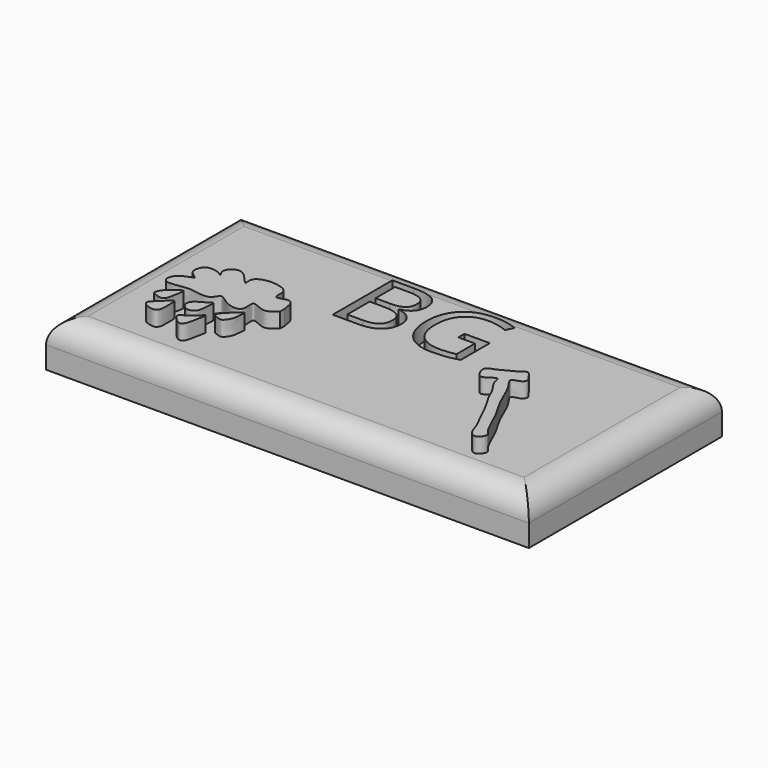
from build123d import *
from build123d import SkipClean  # not in build123d's __all__

# Parameters (mm, degrees)
F0_W         = 101.6
F0_H         = 50.8
F1_DEPTH     = 9.525
F2_TEXT_SIZE = 21.9851628774
F3_DEPTH     = 3.556
F4_T1_DEPTH  = 126.1284097937
F4_T3_DEPTH  = 75.3284097937
F6_DEPTH     = 3.175
F8_DEPTH     = 3.175


# Not quite as in the source:
# - a fillet or chamfer that OpenCascade refuses, or shapes differently, is made with other operations: its cross-section is extruded or revolved along the edge and cut away or added
# - Text() gives the source's letters only with a copy of the font that has no kerning and outlines rounded to 1/6400 em; it was checked with that copy


with BuildPart() as f1:
    # F0 (on Top) → F1 (new body)
    with BuildSketch(Plane.XY):
        with Locations((4.0292814374, -12.5215539605)):
            Rectangle(F0_W, F0_H)
    extrude(amount=F1_DEPTH)

    # F2 (on face) → F3 (cut)
    with BuildSketch(Plane.XY.offset(9.525)):
        with Locations((-12.9512567073, -7.48295011)):
            Text('BG', F2_TEXT_SIZE, font='Open Sans', text_align=(TextAlign.LEFT, TextAlign.BOTTOM))
    extrude(amount=-F3_DEPTH, mode=Mode.SUBTRACT)

    # F4: fillet of radius 4.9056819587 on 4 edges, made by hand

    # F4_s2 → F4_t1 (cut)
    with BuildSketch(Plane.YZ.offset(-59.0349234595)):
        with BuildLine():
            ThreePointArc((-33.0158720017, 9.525), (-36.4847129811, 8.0881590206), (-37.9215539605, 4.6193180413))
            Line((-37.9215539605, 4.6193180413), (-37.9215539605, 9.525))
            Line((-37.9215539605, 9.525), (-33.0158720017, 9.525))
        make_face()
        with BuildLine():
            ThreePointArc((12.8784460395, 4.6193180413), (11.4416050602, 8.0881590206), (7.9727640808, 9.525))
            Line((7.9727640808, 9.525), (12.8784460395, 9.525))
            Line((12.8784460395, 9.525), (12.8784460395, 4.6193180413))
        make_face()
    with SkipClean():  # cleaning this boolean's faces spoils the solid; the shape is the same uncleaned
        extrude(amount=F4_T1_DEPTH, mode=Mode.SUBTRACT)

    # F4_s4 → F4_t3 (cut)
    with BuildSketch(Plane.XZ.offset(-25.1426509364)):
        with BuildLine():
            ThreePointArc((-46.7707185626, 4.6193180413), (-45.3338775832, 8.0881590206), (-41.8650366039, 9.525))
            Line((-41.8650366039, 9.525), (-46.7707185626, 9.525))
            Line((-46.7707185626, 9.525), (-46.7707185626, 4.6193180413))
        make_face()
        with BuildLine():
            ThreePointArc((54.8292814374, 4.6193180413), (53.392440458, 8.0881590206), (49.9235994787, 9.525))
            Line((49.9235994787, 9.525), (54.8292814374, 9.525))
            Line((54.8292814374, 9.525), (54.8292814374, 4.6193180413))
        make_face()
    extrude(amount=F4_T3_DEPTH, mode=Mode.SUBTRACT)

    # F5 (on face) → F6 (join)
    with BuildSketch(Plane.XY.offset(9.525)):
        with BuildLine():
            add(Edge.make_bspline(
                [(-30.1943253726, -12.7980159596), (-30.6638978838, -12.4954709679), (-31.6267253046, -11.8751224446), (-33.7515961581, -11.8213043742), (-34.4176454887, -12.7555614994), (-35.0145429939, -14.6379553372), (-33.6110185049, -15.5878595592), (-32.8381694853, -16.1109231412)],
                knots=[0, 0, 0, 0, 0.2003103356, 0.4107231134, 0.5669213347, 0.7615257699, 1, 1, 1, 1], degree=3))
            add(Edge.make_bspline(
                [(-32.8381694853, -16.1109231412), (-34.112950811, -16.5650307283), (-36.3264014889, -17.3535147812), (-36.5745988024, -20.6952249655), (-32.187577032, -19.7435687353), (-30.2242086338, -19.7475381146), (-26.3365262633, -20.6465069984), (-25.6376160227, -17.6651790254), (-23.2611312044, -20.2929673205), (-18.9913074877, -20.8552925245), (-20.5214901929, -16.0086354704), (-16.807287616, -18.8934549791), (-15.2516189291, -17.4785744542), (-14.4576687431, -16.7564768344)],
                knots=[0, 0, 0, 0, 0.1039781038, 0.1805410855, 0.2831417982, 0.3686725312, 0.4687259635, 0.5411456275, 0.6322911283, 0.7284193522, 0.8168783892, 0.9065421589, 1, 1, 1, 1], degree=3))
            Line((-14.4576687431, -16.7564768344), (-14.4576687431, -15.6208071858))
            add(Edge.make_bspline(
                [(-14.4576687431, -15.6208071858), (-14.6337982566, -14.3014323106), (-14.9696347652, -11.7857025918), (-18.9198891467, -14.113561209), (-17.8391791134, -10.4525662659), (-20.7394672952, -9.4640154529), (-23.252574533, -9.3869308074), (-25.7056960807, -10.5400759818), (-24.7198852466, -13.3743134661), (-27.1734299353, -10.0341195772), (-29.1590570967, -9.1643213191), (-31.2437333359, -11.0235517469), (-30.5359718134, -12.220319388), (-30.1943253726, -12.7980159596)],
                knots=[0, 0, 0, 0, 0.1047918867, 0.1998128573, 0.2885396562, 0.3840489401, 0.4826982162, 0.5732730344, 0.6444100513, 0.7437118311, 0.8326558119, 0.9192206069, 1, 1, 1, 1], degree=3))
        make_face()
        with BuildLine():
            add(Edge.make_bspline(
                [(-22.0946185291, -24.2940131575), (-22.0373505514, -24.6135380633), (-21.0807431356, -24.8821418603), (-19.9589656353, -25.3557262166), (-18.803080228, -23.3856899709), (-18.8393406044, -22.1102220554), (-18.44732324, -20.1385319215), (-20.0988502501, -21.7254314776), (-20.9013918072, -22.4624018961), (-22.1706834832, -23.8696111045), (-22.0946185291, -24.2940131575)],
                knots=[0, 0, 0, 0, 0.1097604899, 0.2172961436, 0.3593928082, 0.4889943909, 0.601999716, 0.726004382, 0.8542130006, 1, 1, 1, 1], degree=3))
        make_face()
        with BuildLine():
            add(Edge.make_bspline(
                [(-23.1663491577, -25.4848245531), (-22.9804289096, -25.5619803766), (-23.5170566685, -27.5027117851), (-23.6440035234, -28.9584264005), (-24.260433732, -30.292487101), (-25.2837995111, -30.384262466), (-27.5699940356, -28.0020978567), (-25.0630939382, -27.6733971885), (-23.3948181393, -25.3900112523), (-23.1663491577, -25.4848245531)],
                knots=[0, 0, 0, 0, 0.1446441433, 0.2900715297, 0.4099252704, 0.5099706331, 0.6753221603, 0.8222533562, 1, 1, 1, 1], degree=3))
        make_face()
        with BuildLine():
            add(Edge.make_bspline(
                [(-24.9525662512, -21.1979039013), (-24.7234080871, -21.3157242906), (-25.0414170545, -23.1626457057), (-25.0353562061, -25.3059194464), (-27.062581453, -25.9756618273), (-28.7073072824, -24.3532164961), (-27.7706908565, -22.6417947192), (-26.221224145, -22.1348562273), (-25.1546234843, -21.0940173043), (-24.9525662512, -21.1979039013)],
                knots=[0, 0, 0, 0, 0.1449106973, 0.3055768692, 0.443566871, 0.5911404454, 0.7260449329, 0.8722268758, 1, 1, 1, 1], degree=3))
        make_face()
        with BuildLine():
            add(Edge.make_bspline(
                [(-30.430296436, -24.6512554586), (-30.1610072747, -24.7340076695), (-30.2245849881, -26.5666013265), (-30.1271662267, -29.4919993977), (-32.7367621761, -28.9792135932), (-34.2156104219, -27.8019858082), (-32.0739136447, -26.247248109), (-30.7275518984, -24.5599092395), (-30.430296436, -24.6512554586)],
                knots=[0, 0, 0, 0, 0.1571543386, 0.3439412931, 0.5106533208, 0.6465377687, 0.8265248205, 1, 1, 1, 1], degree=3))
        make_face()
        with BuildLine():
            add(Edge.make_bspline(
                [(-34.8362959921, -24.2940131575), (-34.7871995093, -24.6206767851), (-33.9812541799, -24.902255674), (-32.4931011173, -25.3854783704), (-31.868783822, -24.3836446627), (-31.6503209763, -22.7748955294), (-31.3306922559, -21.3065937929), (-31.4417532545, -20.6027241278), (-32.5630538646, -21.6052376424), (-33.7740564918, -22.1417022749), (-34.9080176269, -23.8168129992), (-34.8362959921, -24.2940131575)],
                knots=[0, 0, 0, 0, 0.0995996934, 0.2180444325, 0.3129480619, 0.4414438409, 0.5646016246, 0.6249895473, 0.729141728, 0.8545017399, 1, 1, 1, 1], degree=3))
        make_face()
    extrude(amount=F6_DEPTH)

    # F7 (on face) → F8 (join)
    with BuildSketch(Plane.XY.offset(9.525)):
        with BuildLine():
            add(Edge.make_bspline(
                [(24.4670957327, -11.6698769853), (24.6348771213, -11.1302757352), (26.0720557444, -10.893793629), (27.7474509755, -9.7545418913), (29.3142009448, -9.1996198657), (30.9280749843, -7.5848492829), (31.954201958, -9.5784976327), (32.8492776619, -10.366865495), (32.1853787877, -11.652749512), (29.7937320372, -11.7802755298), (31.1561442459, -13.6404811993), (32.0794971607, -15.0675593929), (33.0034144787, -17.3523004539), (34.5916783449, -20.8131512747), (36.0177414598, -22.8321556584), (37.3467899266, -25.952887713), (38.5983209807, -28.6393585317), (40.0393425261, -29.7945368563), (38.4391058362, -31.8989842493), (36.7673079001, -30.6127856865), (36.3253384936, -28.5815760946), (34.8417688599, -25.6772935119), (33.8378756905, -23.6842414053), (32.7427663175, -21.37530851), (31.1768696638, -19.1240104086), (30.5737980965, -16.9284653177), (28.4839321916, -14.565253767), (28.6190150434, -12.4294530929), (26.6631036266, -14.0624038423), (25.2318608541, -14.5495134252), (24.2621768551, -12.3289160089), (24.4670957327, -11.6698769853)],
                knots=[0, 0, 0, 0, 0.0313239544, 0.0657650659, 0.0975737225, 0.1287909347, 0.1603573596, 0.1857324009, 0.2111074332, 0.2425257958, 0.2723768212, 0.3048615766, 0.342408455, 0.3889175923, 0.4270157479, 0.4710245951, 0.5125885033, 0.5418634868, 0.574296285, 0.6041035514, 0.6390900709, 0.6820970547, 0.7182654963, 0.7563154473, 0.7955387388, 0.8319616795, 0.8746153613, 0.9018183914, 0.9344456532, 0.9617426603, 1, 1, 1, 1], degree=3))
        make_face()
    extrude(amount=F8_DEPTH)


solid = f1.part
